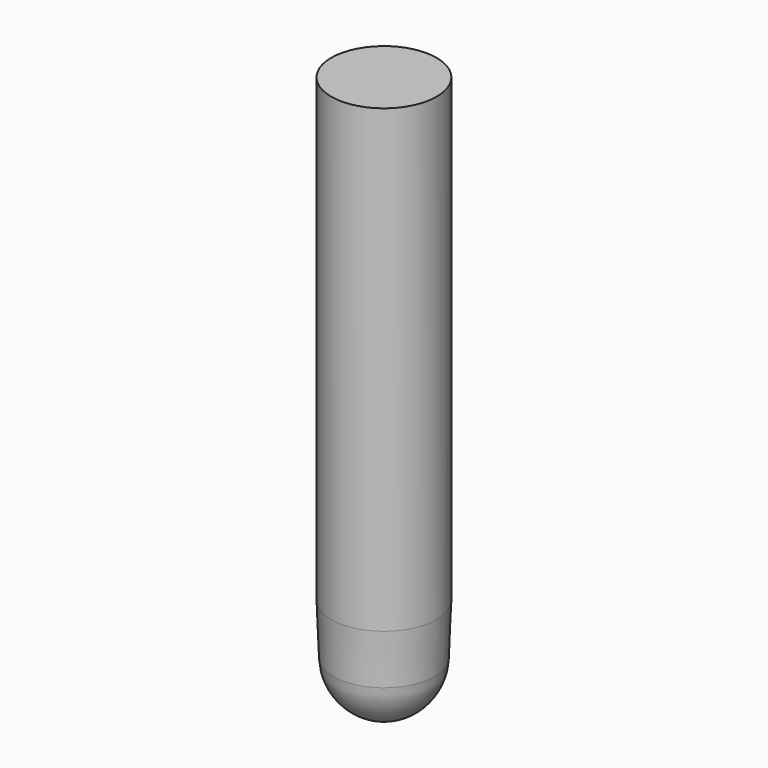
from build123d import *

# Parameters (mm, degrees)
F0_W = 3.267198801
F0_H = 28.5577494651


with BuildPart() as f1:
    # F0 (on Front) → F1 (revolve)
    with BuildSketch(Plane.XZ):
        with BuildLine():
            Line((-57.4008822441, 28.5225976259), (-60.6680810452, 28.5225976259))
            Line((-60.6680810452, 28.5225976259), (-60.547074303, 25.3764055669))
            ThreePointArc((-60.547074303, 25.3764055669), (-59.5904269073, 23.1868609038), (-57.4008822441, 22.230213508))
            Line((-57.4008822441, 22.230213508), (-57.4008822441, 25.3764055669))
            Line((-57.4008822441, 25.3764055669), (-57.4008822441, 28.5225976259))
        make_face()
        with Locations((-59.0344816446, 42.8014723584)):
            Rectangle(F0_W, F0_H)
    revolve(axis=Axis((-57.4008822441, 0, 42.8014723584), (0, 0, -1)))


solid = f1.part
